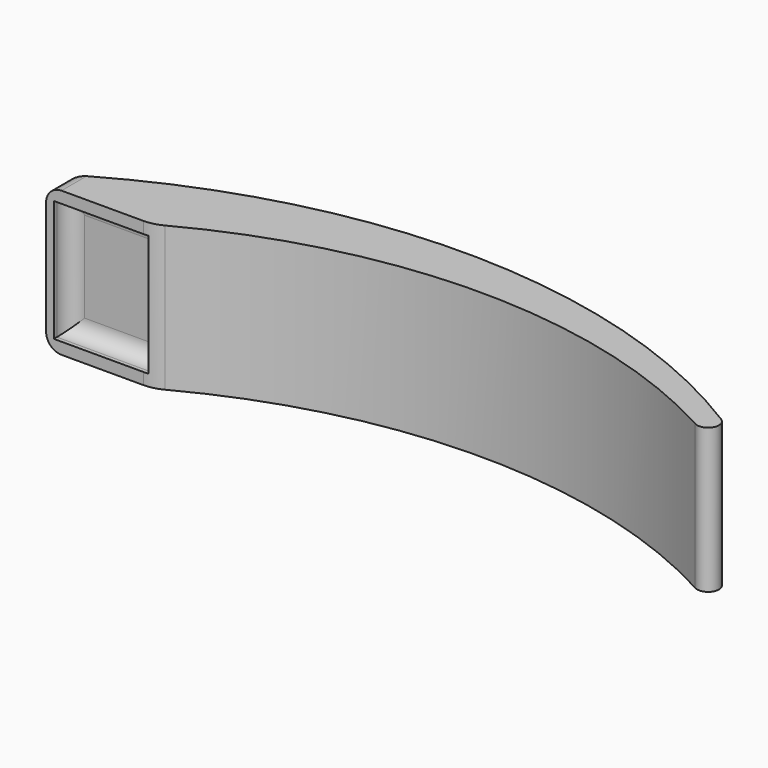
from build123d import *

# Parameters (mm, degrees)
F1_DEPTH    = 7.5
F2_W        = 9.8101310167
F2_H        = 12.6
F3_DEPTH    = 2
F4_R        = 1.6
F5_T1_DEPTH = 20.0711055919


# Not quite as in the source:
# - a fillet or chamfer that OpenCascade refuses, or shapes differently, is made with other operations: its cross-section is extruded or revolved along the edge and cut away or added


with BuildPart() as f1:
    # F0 (on Top) → F1 (new body, symmetric)
    with BuildSketch(Plane.XY):
        with BuildLine():
            ThreePointArc((33.2014997867, 0.1693742672), (34.7428713669, 0.5269798189), (34.3852658153, 2.068351399))
            ThreePointArc((34.3852658153, 2.068351399), (0.2265050268, 11.9077038946), (-34, 2.3066544839))
            Line((-34, 2.3066544839), (-34, 0))
            Line((-34, 0), (-22.8898689833, 0))
            ThreePointArc((-22.8898689833, 0), (5.1340927179, 7.2785489292), (33.2014997867, 0.1693742672))
        make_face()
    extrude(amount=F1_DEPTH, both=True)

    # F2 (on Front) → F3 (cut)
    with BuildSketch(Plane.XZ):
        with Locations((-28.2949344917, 0)):
            Rectangle(F2_W, F2_H)
    extrude(amount=-F3_DEPTH, mode=Mode.SUBTRACT)

    # F4
    f4_edges = [f1.edges().sort_by_distance(p)[0] for p in [
        (-28.294934, 2, 6.3),
        (-33.2, 2, 0),
        (-28.294934, 2, -6.3),
        (-23.389869, 2, 0),
        (-34, 2.306654, 0),
        (-34, 1.153327, 7.5),
        (-34, 1.153327, -7.5),
    ]]
    fillet(f4_edges, radius=F4_R)

    # F5: fillet of radius 4 on 1 edges, made by hand

    # F5_s2 → F5_t1 (cut)
    with BuildSketch(Plane.XY.offset(-10.0355527959)):
        with BuildLine():
            ThreePointArc((-23.9040901017, 0), (-22.9370384998, 0.1186585825), (-22.0273613841, 0.4675944003))
            ThreePointArc((-22.0273613841, 0.4675944003), (-22.4595993901, 0.2356126314), (-22.8898689833, 0))
            Line((-22.8898689833, 0), (-23.9040901017, 0))
        make_face()
    extrude(amount=F5_T1_DEPTH, mode=Mode.SUBTRACT)


solid = f1.part
